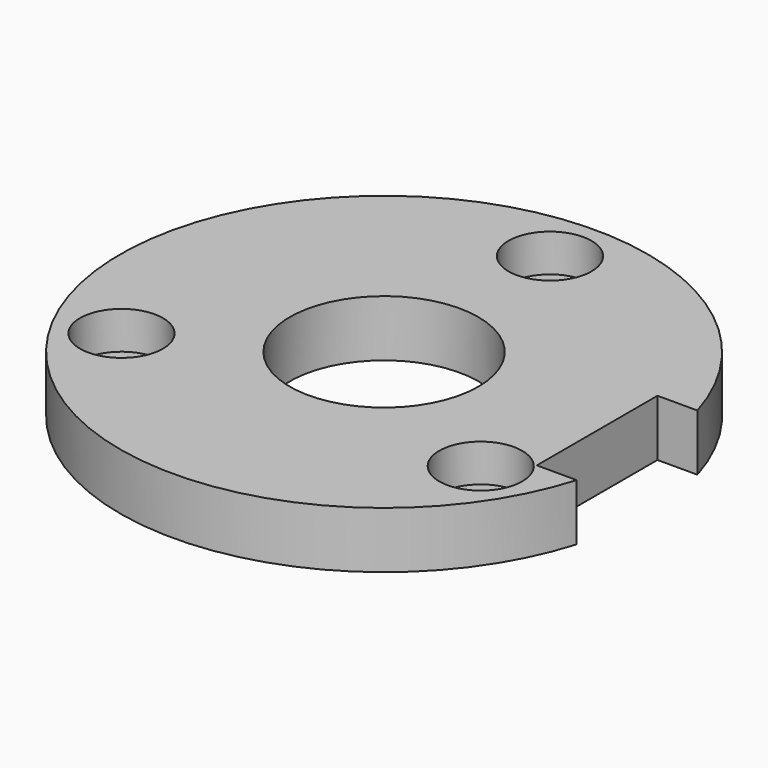
from build123d import *

# Parameters (mm, degrees)
F0_R            = 5
F1_DEPTH        = 3
F3_D            = 2.4
F3_CBORE_D      = 4.4
F3_CBORE_DEPTH  = 2
F3_COPIES_COUNT = 3


# Not quite as in the source:
# - a pattern or mirror of a feature is missing from the dataset's text; its kind, count and spacing are read off the source's solid


with BuildPart() as f1:
    # F0 (on Top) → F1 (new body)
    with BuildSketch(Plane.XY):
        with BuildLine():
            Line((11.3, 4), (13.416407865, 4))
            ThreePointArc((13.416407865, 4), (-14, 0), (13.416407865, -4))
            Line((13.416407865, -4), (11.3, -4))
            Line((11.3, -4), (11.3, 4))
        make_face()
        Circle(F0_R, mode=Mode.SUBTRACT)
    extrude(amount=F1_DEPTH)

    # F3 (through all)
    with Locations(Plane.XY.offset(3)):
        with Locations((0, 11)):
            f3 = CounterBoreHole(F3_D / 2, F3_CBORE_D / 2, F3_CBORE_DEPTH)

    # F3_copies: F3 ×3 about axis
    f3_copies_axis = Axis((0, 0, 0), (0, 0, 1))
    for i in range(1, F3_COPIES_COUNT):
        add(f3.rotate(f3_copies_axis, i * 360 / F3_COPIES_COUNT), mode=Mode.SUBTRACT)


solid = f1.part
